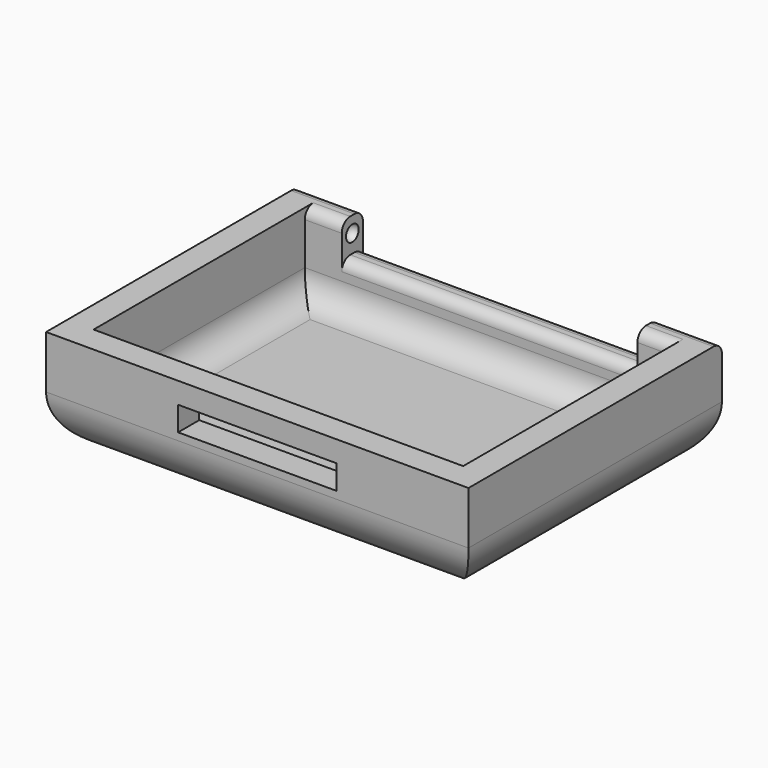
from build123d import *

# Parameters (mm, degrees)
F0_W      = 40
F0_H      = 30
F1_DEPTH  = 10
F2_R      = 5
F3_T      = -2.5
F4_W      = 28
F4_H      = 2.5
F5_DEPTH  = 3
F6_W      = 32.3581136763
F6_H      = 60.2468792349
F7_DEPTH  = 25
F8_R      = 0.75
F9_DEPTH  = 0.75
F10_R     = 0.74999
F11_W     = 14
F11_H     = 2.5
F12_DEPTH = 0.2
F13_R     = 1
F15_W     = 15
F15_H     = 2.3
F16_DEPTH = 2.5


# Not quite as in the source:
# - a fillet or chamfer is up to 0.001 mm smaller than in the source, because OpenCascade refuses the exact size


with BuildPart() as f1:
    # F0 (on Top) → F1 (new body)
    with BuildSketch(Plane.XY):
        Rectangle(F0_W, F0_H)
    extrude(amount=-F1_DEPTH)

    # F2
    f2_edges = [f1.edges().sort_by_distance(p)[0] for p in [
        (20, 0, -10),
        (0, 15, -10),
        (-20, 0, -10),
        (0, -15, -10),
    ]]
    fillet(f2_edges, radius=F2_R)

    # F3
    f3_openings = [f1.faces().sort_by_distance(p)[0] for p in [
        (0, 0, 0),
    ]]
    offset(amount=F3_T, openings=f3_openings)

    # F4 (on face) → F5 (cut)
    with BuildSketch(Plane.XY):
        with Locations((0, 13.75)):
            Rectangle(F4_W, F4_H)
    extrude(amount=-F5_DEPTH, mode=Mode.SUBTRACT)

    # F6 (on Top) → F7 (cut)
    with BuildSketch(Plane.XY):
        with Locations((16.1790568382, -2.0559011027)):
            Rectangle(F6_W, F6_H)
    extrude(amount=-F7_DEPTH, mode=Mode.SUBTRACT)

    # F8 (on face) → F9 (cut)
    with BuildSketch(Plane.YZ.offset(-14)):
        with Locations((13.75, -1.5)):
            Circle(F8_R)
    extrude(amount=-F9_DEPTH, mode=Mode.SUBTRACT)

    # F10 (radius 0.75 in the source; OpenCascade refuses exactly that, so slightly less here)
    f10_edges = [f1.edges().sort_by_distance(p)[0] for p in [
        (-14.75, 13, -1.5),
    ]]
    fillet(f10_edges, radius=F10_R)

    # F11 (on face) → F12 (cut)
    with BuildSketch(Plane.XY.offset(-3)):
        with Locations((-7, 13.75)):
            Rectangle(F11_W, F11_H)
    extrude(amount=-F12_DEPTH, mode=Mode.SUBTRACT)

    # F13
    f13_edges = [f1.edges().sort_by_distance(p)[0] for p in [
        (-17, 15, 0),
        (-15.75, 12.5, 0),
        (-7, 15, -3.2),
        (-7, 12.5, -3.2),
    ]]
    fillet(f13_edges, radius=F13_R)

    # F14: F1 across plane


with BuildPart() as f1_1:
    add(f1.part)
    add(f1.part.mirror(Plane.YZ))

    # F15 (on face) → F16 (cut, through all)
    with BuildSketch(Plane.XZ.offset(15)):
        with Locations((0, -3.15)):
            Rectangle(F15_W, F15_H)
    extrude(amount=-F16_DEPTH, mode=Mode.SUBTRACT)


solid = f1_1.part
